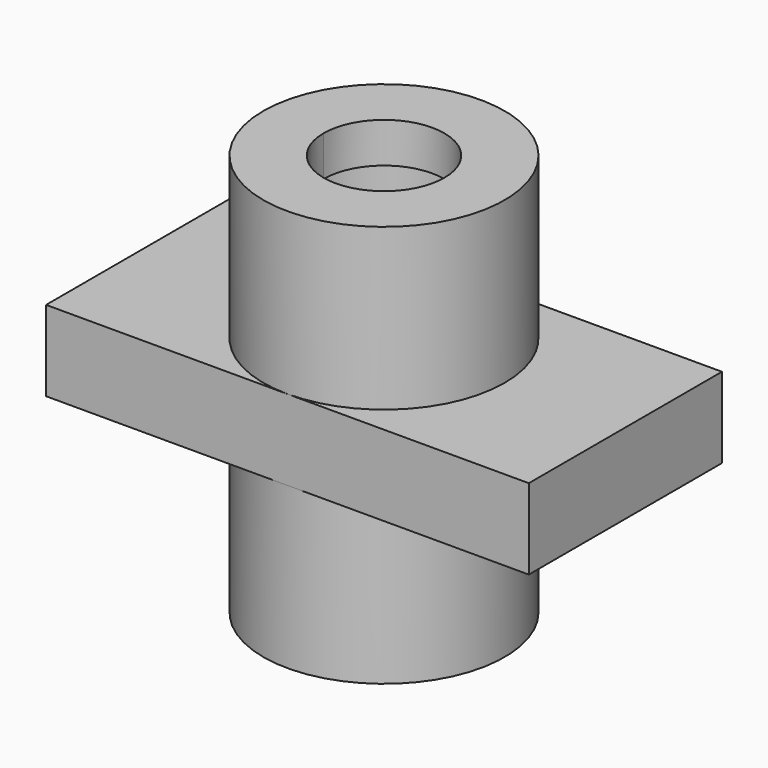
from build123d import *
from build123d import SkipClean  # not in build123d's __all__

# Parameters (mm, degrees)
F2_W     = 76.2
F2_H     = 38.1
F3_DEPTH = 6.35
F4_R     = 9.525
F5_DEPTH = 63.501


with BuildPart() as f1:
    # F0 (on Front) → F1 (revolve)
    with BuildSketch(Plane.XZ):
        Polygon((-9.525, 25.4), (-9.525, 31.75), (-19.05, 31.75), (-19.05, -31.75), (-9.525, -31.75), (-9.525, 19.05), (-12.7, 19.05), (-12.7, 25.4), align=None)
    revolve(axis=Axis((0, 0, 1.6377754509), (0, 0, -1)))

    # F2 (on Top) → F3 (join, symmetric)
    with BuildSketch(Plane.XY):
        Rectangle(F2_W, F2_H)
    extrude(amount=F3_DEPTH, both=True)

    # F4 (on face) → F5 (cut, through all)
    with BuildSketch(Plane.XY.offset(31.75)):
        Circle(F4_R)
    with SkipClean():  # cleaning this boolean's faces spoils the solid; the shape is the same uncleaned
        extrude(amount=-F5_DEPTH, mode=Mode.SUBTRACT)


solid = f1.part
